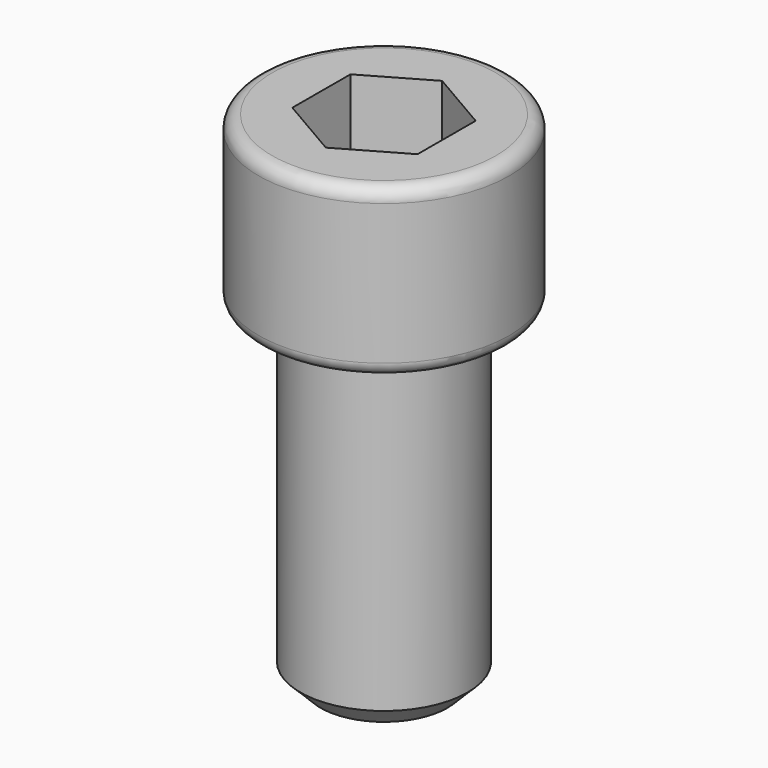
from build123d import *

# Parameters (mm, degrees)
F0_R     = 3.175
F1_DEPTH = 12.7
F2_R     = 4.7625
F2_R_2   = 3.175
F3_DEPTH = 6.35
F5_DEPTH = 4.826
F6_SIZE2 = 0.762
F6_SIZE  = 0.762
F10_R    = 0.508


# Not quite as in the source:
# - the program builds the solid bodies; features that only make, move or delete a surface that nothing else refers to are left out


with BuildPart() as f1:
    # F0 (on Top) → F1 (new body)
    with BuildSketch(Plane.XY):
        with Locations((-48.0243302882, -37.1180400252)):
            Circle(F0_R)
    extrude(amount=-F1_DEPTH)

    # F2 (on Top) → F3 (join)
    with BuildSketch(Plane.XY):
        with Locations((-48.0243302882, -37.1180400252)):
            Circle(F2_R)
        with Locations((-48.0243302882, -37.1180400252)):
            Circle(F2_R_2, mode=Mode.SUBTRACT)
        with Locations((-48.0243302882, -37.1180400252)):
            Circle(F2_R_2)
    extrude(amount=F3_DEPTH)

    # F4 (on face) → F5 (cut)
    with BuildSketch(Plane.XY.offset(6.35)):
        Polygon((-48.016363853, -34.3684209087), (-50.4015870762, -35.7363313317), (-50.4095535114, -38.4859504482), (-48.0322967234, -39.8676591418), (-45.6470735001, -38.4997487188), (-45.6391070649, -35.7501296023), align=None)
    extrude(amount=-F5_DEPTH, mode=Mode.SUBTRACT)

    # F6
    f6_edges = [f1.edges().sort_by_distance(p)[0] for p in [
        (-51.19933, -37.11804, -12.7),
    ]]
    chamfer(f6_edges, length=F6_SIZE, length2=F6_SIZE2)

    # F10
    f10_edges = [f1.edges().sort_by_distance(p)[0] for p in [
        (-52.78683, -37.11804, 0),
        (-52.78683, -37.11804, 6.35),
    ]]
    fillet(f10_edges, radius=F10_R)


solid = f1.part
